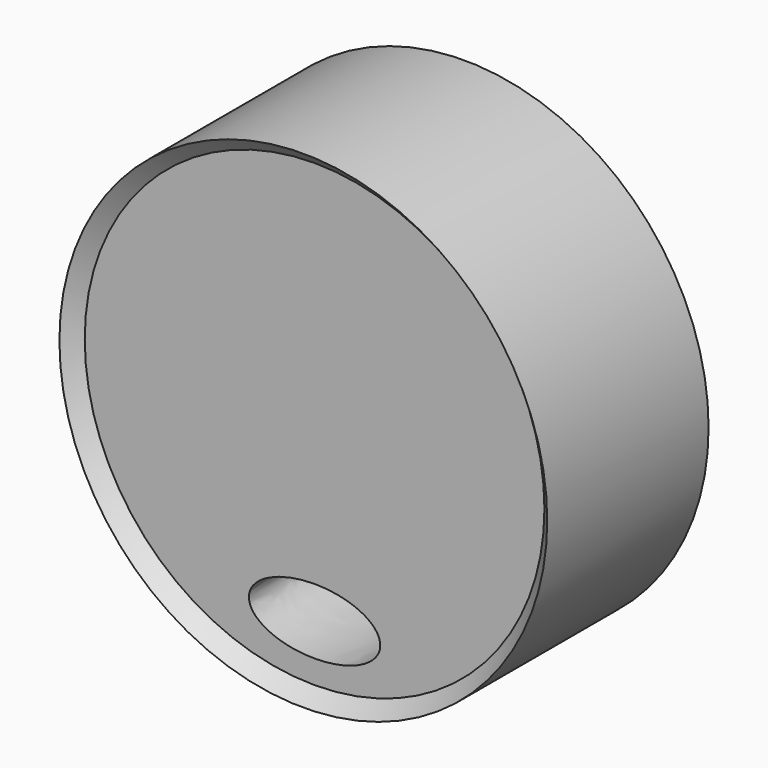
from build123d import *

# Parameters (mm, degrees)
F0_R     = 33.02
F0_R_2   = 28.575
F1_DEPTH = 27.94
F2_DEPTH = 25.4


# Not quite as in the source:
# - a fillet or chamfer that OpenCascade refuses, or shapes differently, is made with other operations: its cross-section is extruded or revolved along the edge and cut away or added


with BuildPart() as f1:
    # F0 (on Front) → F1 (new body)
    with BuildSketch(Plane.XZ):
        Circle(F0_R)
        Circle(F0_R_2, mode=Mode.SUBTRACT)
    extrude(amount=F1_DEPTH)

    # F0 (on Front) → F2 (join)
    with BuildSketch(Plane.XZ):
        Circle(F0_R_2)
        with BuildLine():
            add(Edge.make_bspline(
                [(-8.89, -23.495), (-8.89, -31.1939658396), (4.445, -27.3444829198), (17.78, -23.495), (4.445, -19.6455170802), (-8.89, -15.7960341604), (-8.89, -23.495)],
                knots=[0, 0, 0, 2.0943951024, 2.0943951024, 4.1887902048, 4.1887902048, 6.2831853072, 6.2831853072, 6.2831853072], degree=2, weights=[1, 0.5, 1, 0.5, 1, 0.5, 1]))
        make_face(mode=Mode.SUBTRACT)
    extrude(amount=F2_DEPTH)

    # F3: chamfer of 5.08 on 1 edges, made by hand


with BuildPart() as f3_tool2:
    # F3_s3 → F3_t4 (revolve)
    with BuildSketch(Plane.XY):
        Polygon((33.655, -27.94), (28.575, -22.86), (28.575, -27.94), align=None)
    revolve(axis=Axis((0, -27.94, 0), (0, -1, 0)))

    split(bisect_by=Plane.XZ.offset(25.4), keep=Keep.TOP)


with BuildPart() as f1_1:
    add(f1.part)

    # F3_t1: cut F3_tool2
    add(f3_tool2.part, mode=Mode.SUBTRACT)


solid = f1_1.part
